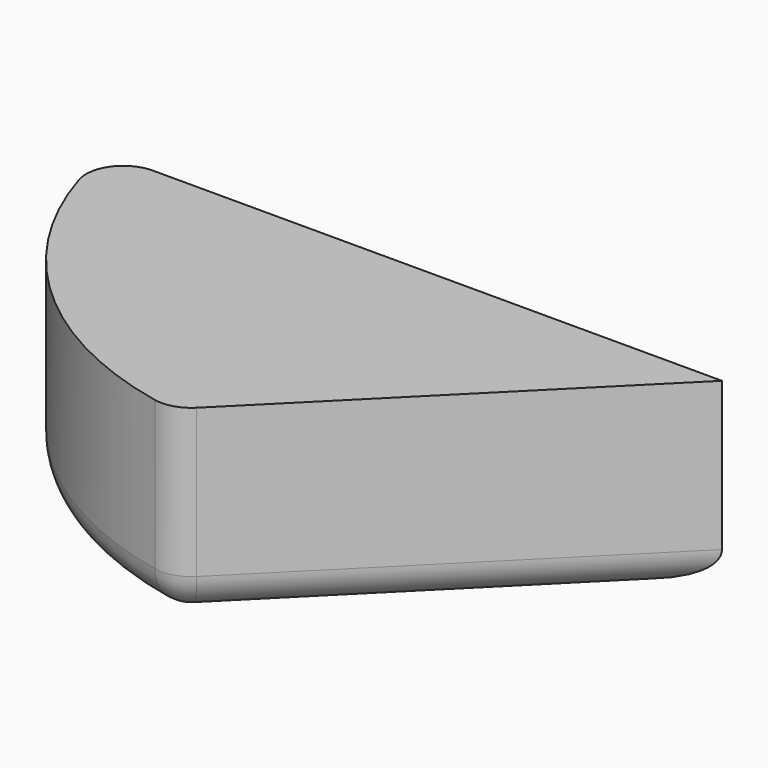
from build123d import *

# Parameters (mm, degrees)
F0_W        = 118.0765684694
F0_H        = 42.3587011173
F1_DEPTH    = 25.4
F2_T1_DEPTH = 275.8687841416
F3_T1_DEPTH = 417.324487366
F4_R        = 5.08
F5_T1_DEPTH = 59.2305880834
F6_R        = 5.08


# Not quite as in the source:
# - a fillet or chamfer that OpenCascade refuses, or shapes differently, is made with other operations: its cross-section is extruded or revolved along the edge and cut away or added


with BuildPart() as f1:
    # F0 (on Top) → F1 (new body)
    with BuildSketch(Plane.XY):
        with Locations((-49.8337792233, -36.1952199601)):
            Rectangle(F0_W, F0_H)
    extrude(amount=F1_DEPTH)

    # F2: fillet of radius 50.8 on 1 edges, made by hand

    # F2_s2 → F2_t1 (cut)
    with BuildSketch(Plane.XY.offset(-125.2343920708)):
        with BuildLine():
            ThreePointArc((-108.872063458, -15.0158694014), (-91.5793890566, -45.3654069575), (-58.7783066297, -57.3745705187))
            Line((-58.7783066297, -57.3745705187), (-108.872063458, -57.3745705187))
            Line((-108.872063458, -57.3745705187), (-108.872063458, -15.0158694014))
        make_face()
    extrude(amount=F2_T1_DEPTH, mode=Mode.SUBTRACT)

    # F3: chamfer of 76.2 on 1 edges, made by hand

    # F3_s2 → F3_t1 (cut)
    with BuildSketch(Plane.XY.offset(-195.962243683)):
        Polygon((9.2045050114, 18.8254294813), (-66.9954949886, -57.3745705187), (9.2045050114, -57.3745705187), align=None)
    extrude(amount=F3_T1_DEPTH, mode=Mode.SUBTRACT)

    # F4
    f4_edges = [f1.edges().sort_by_distance(p)[0] for p in [
        (-66.417785, -56.79686, 12.7),
    ]]
    fillet(f4_edges, radius=F4_R)

    # F5: fillet of radius 5.08 on 1 edges, made by hand

    # F5_s2 → F5_t1 (cut)
    with BuildSketch(Plane.XY.offset(-16.9152940417)):
        with BuildLine():
            ThreePointArc((-102.4531606824, -15.0158694014), (-106.5420738654, -17.081372929), (-107.3059222438, -21.5982359439))
            ThreePointArc((-107.3059222438, -21.5982359439), (-108.1987038654, -18.3331561934), (-108.872063458, -15.0158694014))
            Line((-108.872063458, -15.0158694014), (-102.4531606824, -15.0158694014))
        make_face()
    extrude(amount=F5_T1_DEPTH, mode=Mode.SUBTRACT)

    # F6
    f6_edges = [f1.edges().sort_by_distance(p)[0] for p in [
        (-44.588616, -34.967691, 0),
        (-66.681498, -56.195765, 0),
        (-92.968648, -44.146642, 0),
        (-106.542074, -17.081373, 0),
        (-63.544977, -15.015869, 0),
    ]]
    fillet(f6_edges, radius=F6_R)


solid = f1.part
